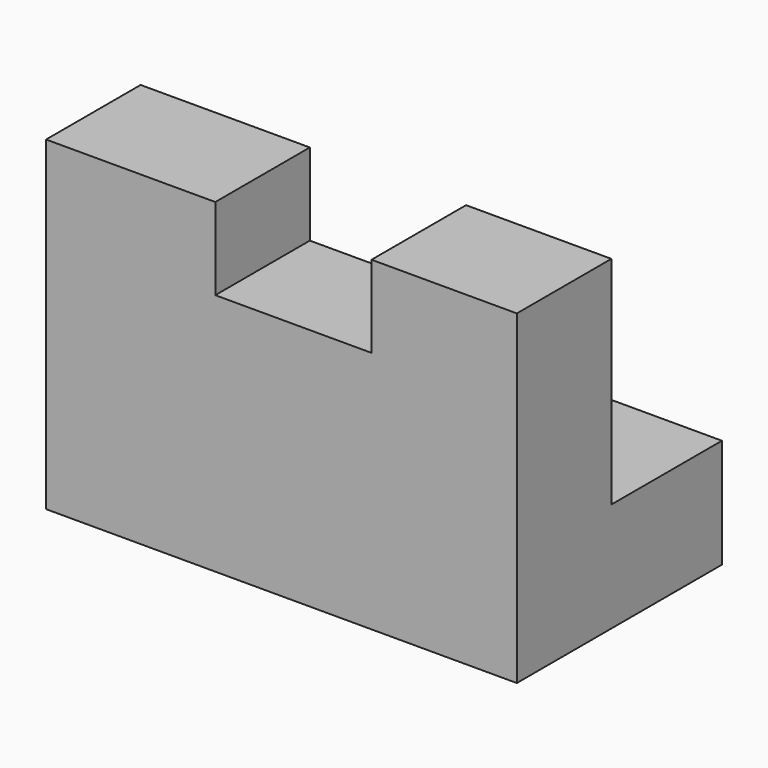
from build123d import *

# Parameters (mm, degrees)
F1_DEPTH = 72.898
F2_W     = 24.1890717298
F2_H     = 18.2968638837
F3_DEPTH = 12.7


# Not quite as in the source:
# - a length typed as a fraction of an inch, garbled in the dataset ("3 / 203.2 mm" for 3/8 in), is restored


with BuildPart() as f1:
    # F0 (on Right) → F1 (new body)
    with BuildSketch(Plane.YZ):
        Polygon((-3.8764555939, 0), (0, 0), (6.0472693294, 0), (6.0472693294, 16.9013366103), (-15.3507553041, 16.9013366103), (-15.3507553041, 50.3938943148), (-33.6476191878, 50.3938943148), (-33.6476191878, 0), align=None)
    extrude(amount=F1_DEPTH)

    # F2 (on face) → F3 (cut)
    with BuildSketch(Plane.XY.offset(50.3938943148)):
        with Locations((38.2993584499, -24.499187246)):
            Rectangle(F2_W, F2_H)
    extrude(amount=-F3_DEPTH, mode=Mode.SUBTRACT)


solid = f1.part
